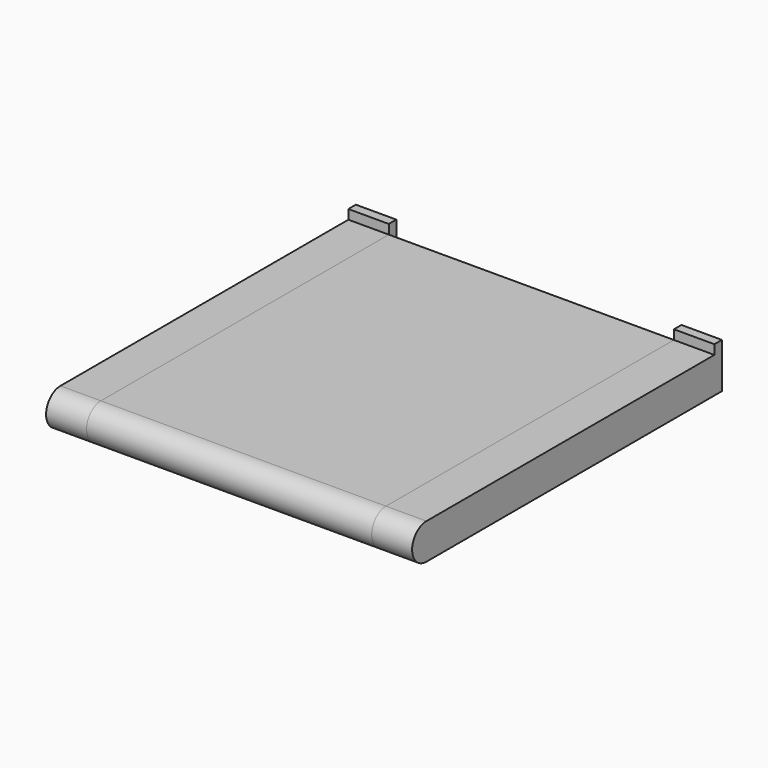
from build123d import *

# Parameters (mm, degrees)
F0_W      = 8.6
F0_H      = 78.5
F1_DEPTH  = 7.6
F3_DEPTH  = 8.6
F4_W      = 8.6
F4_H      = 2
F5_DEPTH  = 2
F6_R      = 3.225
F7_DEPTH  = 30.3
F9_W      = 60.6
F9_H      = 76.5
F10_DEPTH = 7.6
F12_DEPTH = 60.6
F14_R     = 2.6
F15_DEPTH = 60.6


# Not quite as in the source:
# - a feature names something its author has since deleted; it is built from what else it names


with BuildPart() as f1:
    # F0 (on Top) → F1 (new body)
    with BuildSketch(Plane.XY):
        with Locations((-34.6, 0)):
            Rectangle(F0_W, F0_H)
    extrude(amount=F1_DEPTH)

    # F2 (on face) → F3 (join)
    with BuildSketch(Plane(origin=(-38.9, 0, 0), x_dir=(0, -1, 0), z_dir=(-1, 0, 0))):
        with BuildLine():
            Line((39.25, 7.6), (39.25, 0))
            ThreePointArc((39.25, 0), (43.05, 3.8), (39.25, 7.6))
        make_face()
    extrude(amount=-F3_DEPTH)

    # F4 (on face) → F5 (join)
    with BuildSketch(Plane.XY.offset(7.6)):
        with Locations((-34.6, 38.25)):
            Rectangle(F4_W, F4_H)
    extrude(amount=F5_DEPTH)

    # F6 (on face) → F7 (join)
    with BuildSketch(Plane.YZ.offset(-30.3)):
        with Locations((-22.45, 3.8)):
            Circle(F6_R)
    extrude(amount=F7_DEPTH)

    # F8: F1 across plane


with BuildPart() as f1_1:
    add(f1.part)
    add(f1.part.mirror(Plane.YZ))


with BuildPart() as f10:
    # F9 (on face) → F10 (new body)
    with BuildSketch(Plane.XY.offset(7.6)):
        with Locations((0, -1)):
            Rectangle(F9_W, F9_H)
    extrude(amount=-F10_DEPTH)


with BuildPart() as f12:
    # F11 (on face) → F12 (new body)
    with BuildSketch(Plane(origin=(-30.3, 0, 0), x_dir=(0, -1, 0), z_dir=(-1, 0, 0))):
        with BuildLine():
            Line((39.25, 7.6), (39.25, 0))
            ThreePointArc((39.25, 0), (43.05, 3.8), (39.25, 7.6))
        make_face()
    extrude(amount=-F12_DEPTH)

    # F13: union F10
    add(f10.part)

    # F14 (on face) → F15 (cut)
    with BuildSketch(Plane.YZ.offset(30.3)):
        with Locations((20.05, 3.8)):
            Circle(F14_R)
    extrude(amount=-F15_DEPTH, mode=Mode.SUBTRACT)

    # F17: cut F1
    add(f1_1.part, mode=Mode.SUBTRACT)


solid = Compound([f1_1.part, f12.part])
